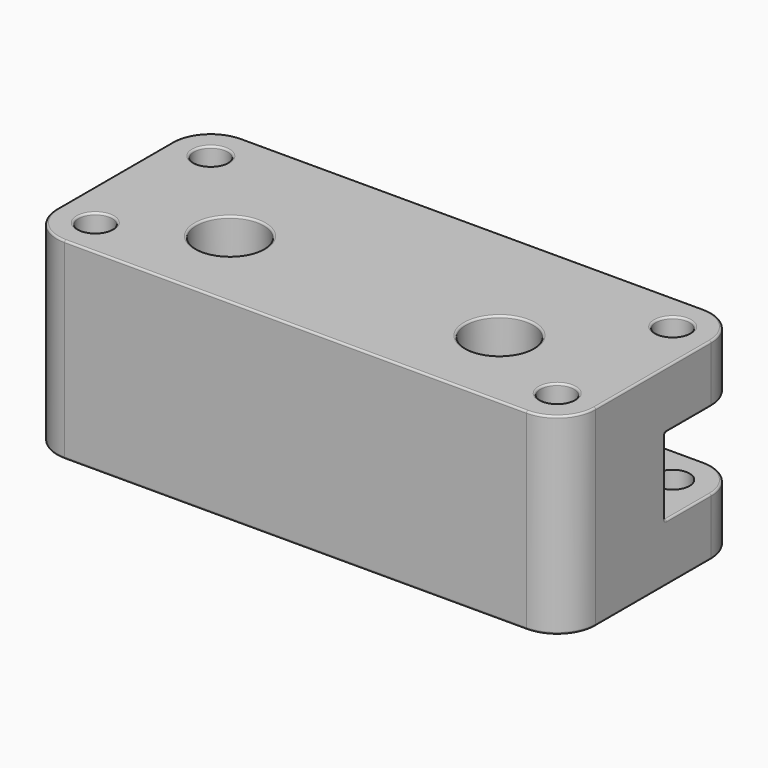
from build123d import *

# Parameters (mm, degrees)
F0_W     = 56
F0_H     = 15
F0_R     = 1.75
F0_H_2   = 8
F1_DEPTH = 10
F2_R     = 3.5
F3_DEPTH = 5
F5_R     = 4
F4_W     = 10
F4_H     = 8
F6_DEPTH = 56.001
F7_R     = 1.75
F8_DEPTH = 15
F9_R     = 0.2


# Not quite as in the source:
# - a feature names something its author has since deleted; it is built from what else it names


with BuildPart() as f1:
    # F0 (on Top) → F1 (new body, symmetric)
    with BuildSketch(Plane.XY):
        with Locations((0, 7.5)):
            Rectangle(F0_W, F0_H)
        with Locations((-24, 4)):
            Circle(F0_R, mode=Mode.SUBTRACT)
        with Locations((24, 4)):
            Circle(F0_R, mode=Mode.SUBTRACT)
        with Locations((0, 19)):
            Rectangle(F0_W, F0_H_2)
        with Locations((-24, 19)):
            Circle(F0_R, mode=Mode.SUBTRACT)
        with Locations((24, 19)):
            Circle(F0_R, mode=Mode.SUBTRACT)
    extrude(amount=F1_DEPTH, both=True)

    # F2 (on face) → F3 (cut)
    with BuildSketch(Plane.XY.offset(10)):
        with Locations((-14, 9)):
            Circle(F2_R)
        with Locations((14, 9)):
            Circle(F2_R)
    extrude(amount=-F3_DEPTH, mode=Mode.SUBTRACT)

    # F5
    f5_edges = [f1.edges().sort_by_distance(p)[0] for p in [
        (-28, 23, 0),
        (28, 23, 0),
        (-28, 0, 0),
        (28, 0, 0),
    ]]
    fillet(f5_edges, radius=F5_R)

    # F4 (on face) → F6 (cut, through all)
    with BuildSketch(Plane(origin=(-28, 0, 0), x_dir=(0, -1, 0), z_dir=(-1, 0, 0))):
        with Locations((-18, 0)):
            Rectangle(F4_W, F4_H)
    extrude(amount=-F6_DEPTH, mode=Mode.SUBTRACT)

    # F7 (on face) → F8 (cut)
    with BuildSketch(Plane(origin=(0, 0, -10), x_dir=(1, 0, 0), z_dir=(0, 0, -1))):
        with BuildLine():
            ThreePointArc((24, -7.25), (22.7625631329, -10.2374368671), (25.75, -9))
            ThreePointArc((25.75, -9), (25.2374368671, -7.7625631329), (24, -7.25))
        make_face()
        with Locations((-24, -9)):
            Circle(F7_R)
    extrude(amount=-F8_DEPTH, mode=Mode.SUBTRACT)

    # F9
    f9_edges = [f1.edges().sort_by_distance(p)[0] for p in [
        (0, 0, 10),
        (-26.828427, 1.171573, 10),
        (26.828427, 1.171573, 10),
        (-28, 11.5, 10),
        (28, 11.5, 10),
        (-26.828427, 21.828427, 10),
        (26.828427, 21.828427, 10),
        (0, 23, 10),
        (-25.75, 4, 10),
        (-17.5, 9, 10),
        (22.25, 4, 10),
        (10.5, 9, 10),
        (-25.75, 19, 10),
        (22.25, 19, 10),
        (-28, 19, -7),
        (-28, 16, -4),
        (-28, 13, 0),
        (-28, 16, 4),
        (-28, 19, 7),
        (-28, 4, 0),
        (-28, 11.5, -10),
        (0, 0, -10),
        (-26.828427, 1.171573, -10),
        (26.828427, 1.171573, -10),
        (28, 11.5, -10),
        (-26.828427, 21.828427, -10),
        (26.828427, 21.828427, -10),
        (0, 23, -10),
        (-25.75, 4, -10),
        (-25.75, 9, -10),
        (22.25, 4, -10),
        (22.25, 9, -10),
        (-25.75, 19, -10),
        (22.25, 19, -10),
        (0, 13, 4),
        (28, 13, 0),
        (0, 13, -4),
    ]]
    fillet(f9_edges, radius=F9_R)


solid = f1.part
